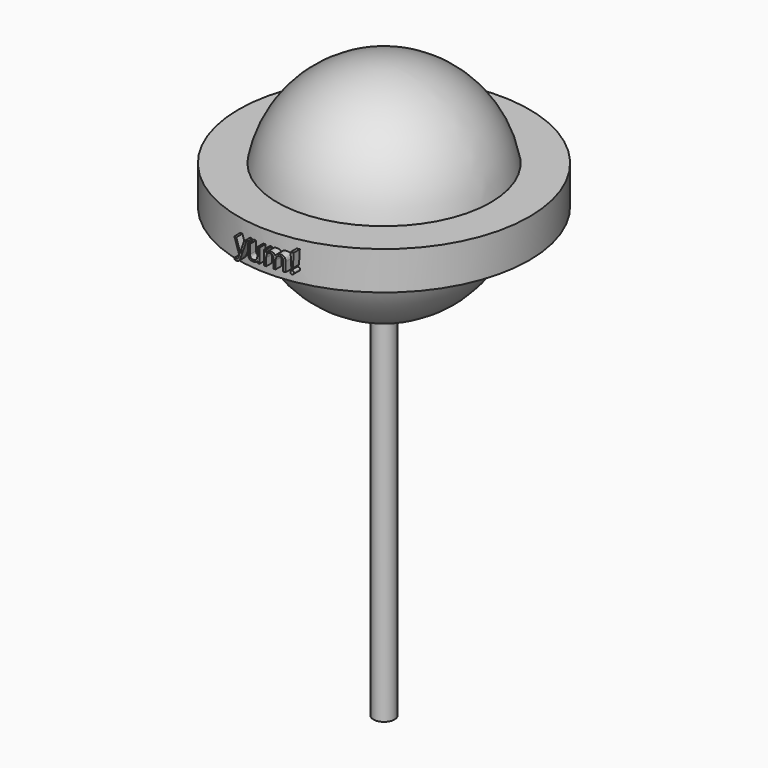
from build123d import *

# Parameters (mm, degrees)
F2_TEXT_SIZE = 5.2916666667
F3_DEPTH     = 31.75


# Not quite as in the source:
# - Text() gives the source's letters only with a copy of the font that has no kerning and outlines rounded to 1/6400 em; it was checked with that copy


with BuildPart() as f1:
    # F0 (on Front) → F1 (revolve)
    with BuildSketch(Plane.XZ):
        with BuildLine():
            Line((0, -17.185240984), (0, -21.59))
            ThreePointArc((0, -21.59), (1.0485396886, -21.5645232853), (2.0946047734, -21.4881532674))
            Line((2.0946047734, -21.4881532674), (2.0946047734, -17.185240984))
            Line((2.0946047734, -17.185240984), (0, -17.185240984))
        make_face()
        with BuildLine():
            ThreePointArc((2.0946047734, -21.4881532674), (1.0485396886, -21.5645232853), (0, -21.59))
            Line((0, -21.59), (0, -93.0868163705))
            Line((0, -93.0868163705), (2.0946047734, -93.0868163705))
            Line((2.0946047734, -93.0868163705), (2.0946047734, -21.4881532674))
        make_face()
        with BuildLine():
            Line((2.0946047734, -17.185240984), (2.0946047734, -21.4881532674))
            ThreePointArc((2.0946047734, -21.4881532674), (14.6419094375, -15.8663980797), (21.2511646488, -3.8100001402))
            Line((21.2511646488, -3.8100001402), (5.7912003249, -3.8100001402))
            Line((5.7912003249, -3.8100001402), (5.7912003249, 3.8100001402))
            Line((5.7912003249, 3.8100001402), (21.2511646488, 3.8100001402))
            ThreePointArc((21.2511646488, 3.8100001402), (13.854064331, 16.5587741549), (0, 21.59))
            Line((0, 21.59), (0, -17.185240984))
            Line((0, -17.185240984), (2.0946047734, -17.185240984))
        make_face()
        with BuildLine():
            Line((5.7912003249, -3.8100001402), (21.2511646488, -3.8100001402))
            ThreePointArc((21.2511646488, -3.8100001402), (21.59, 0), (21.2511646488, 3.8100001402))
            Line((21.2511646488, 3.8100001402), (5.7912003249, 3.8100001402))
            Line((5.7912003249, 3.8100001402), (5.7912003249, -3.8100001402))
        make_face()
        with BuildLine():
            ThreePointArc((21.2511646488, 3.8100001402), (21.59, 0), (21.2511646488, -3.8100001402))
            Line((21.2511646488, -3.8100001402), (28.9560053498, -3.8100001402))
            Line((28.9560053498, -3.8100001402), (28.9560053498, 3.8100001402))
            Line((28.9560053498, 3.8100001402), (21.2511646488, 3.8100001402))
        make_face()
    revolve(axis=Axis((0, 0, 24.1554006934), (0, 0, 1)))

    # F2 (on Front) → F3 (join)
    with BuildSketch(Plane.XZ):
        with Locations((-5.9050807965, -1.6252210412)):
            Text('yum!', F2_TEXT_SIZE, font='Open Sans', text_align=(TextAlign.LEFT, TextAlign.BOTTOM))
    extrude(amount=F3_DEPTH)

    # F4 (on Front) → F5 (revolve, cut)
    with BuildSketch(Plane.XZ):
        Polygon((30.4560053498, 5.3100001402), (30.4560053498, -5.3100001402), (25.04003793, -5.3100001402), (26.4452621341, -11.8494375944), (40.6536348164, -11.8494375944), (40.6536348164, 10.0135614499), (31.2854759395, 12.5898055136), (18.7945980579, 11.5749209523), (21.3708411902, 5.3100001402), align=None)
    revolve(axis=Axis((0, 0, 27.5195743889), (0, 0, 1)), mode=Mode.SUBTRACT)


solid = f1.part
